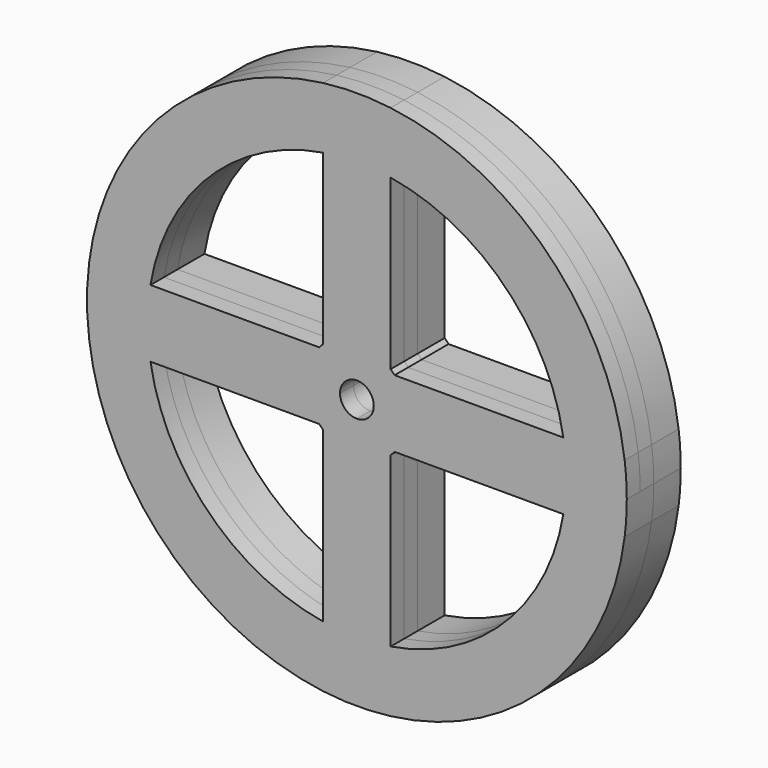
from build123d import *

# Parameters (mm, degrees)
F1_DEPTH = 2.5
F2_DEPTH = 5


# Not quite as in the source:
# - a feature names something its author has since deleted; it is built from what else it names


with BuildPart() as f1:
    # F0 (on Front) → F1 (new body, symmetric)
    with BuildSketch(Plane.XZ):
        with BuildLine():
            ThreePointArc((39.686269666, -5), (39.9214903695, -2.5049165017), (40, 0))
            ThreePointArc((40, 0), (39.9214903695, 2.5049165017), (39.686269666, 5))
            ThreePointArc((39.686269666, 5), (28.2842712475, 28.2842712475), (5, 39.686269666))
            ThreePointArc((5, 39.686269666), (0, 40), (-5, 39.686269666))
            ThreePointArc((-5, 39.686269666), (-28.2842712475, 28.2842712475), (-39.686269666, 5))
            ThreePointArc((-39.686269666, 5), (-40, 0), (-39.686269666, -5))
            ThreePointArc((-39.686269666, -5), (-28.2842712475, -28.2842712475), (-5, -39.686269666))
            ThreePointArc((-5, -39.686269666), (0, -40), (5, -39.686269666))
            ThreePointArc((5, -39.686269666), (28.2842712475, -28.2842712475), (39.686269666, -5))
        make_face()
        with BuildLine():
            ThreePointArc((30.5941170816, 5), (30.8983626551, 2.5082235219), (31, 0))
            ThreePointArc((31, 0), (30.8983626551, -2.5082235219), (30.5941170816, -5))
            ThreePointArc((30.5941170816, -5), (21.9203102168, -21.9203102168), (5, -30.5941170816))
            ThreePointArc((5, -30.5941170816), (2.5082235219, -30.8983626551), (0, -31))
            ThreePointArc((0, -31), (-2.5082235219, -30.8983626551), (-5, -30.5941170816))
            ThreePointArc((-5, -30.5941170816), (-21.9203102168, -21.9203102168), (-30.5941170816, -5))
            ThreePointArc((-30.5941170816, -5), (-30.8983626551, -2.5082235219), (-31, 0))
            ThreePointArc((-31, 0), (-30.8983626551, 2.5082235219), (-30.5941170816, 5))
            ThreePointArc((-30.5941170816, 5), (-21.9203102168, 21.9203102168), (-5, 30.5941170816))
            ThreePointArc((-5, 30.5941170816), (-2.5082235219, 30.8983626551), (0, 31))
            ThreePointArc((0, 31), (2.5082235219, 30.8983626551), (5, 30.5941170816))
            ThreePointArc((5, 30.5941170816), (21.9203102168, 21.9203102168), (30.5941170816, 5))
        make_face(mode=Mode.SUBTRACT)
        with BuildLine():
            Line((7.5, 0), (31, 0))
            ThreePointArc((31, 0), (30.8983626551, 2.5082235219), (30.5941170816, 5))
            Line((30.5941170816, 5), (5.5901699437, 5))
            ThreePointArc((5.5901699437, 5), (7.0062926922, 2.6761656733), (7.5, 0))
        make_face()
        with BuildLine():
            ThreePointArc((30.5941170816, -5), (30.8983626551, -2.5082235219), (31, 0))
            Line((31, 0), (7.5, 0))
            ThreePointArc((7.5, 0), (7.0062926922, -2.6761656733), (5.5901699437, -5))
            Line((5.5901699437, -5), (30.5941170816, -5))
        make_face()
        with BuildLine():
            Line((2.5, 0), (7.5, 0))
            ThreePointArc((7.5, 0), (7.0062926922, 2.6761656733), (5.5901699437, 5))
            ThreePointArc((5.5901699437, 5), (5.3033008589, 5.3033008589), (5, 5.5901699437))
            ThreePointArc((5, 5.5901699437), (2.6761656733, 7.0062926922), (0, 7.5))
            Line((0, 7.5), (0, 2.5))
            ThreePointArc((0, 2.5), (1.767766953, 1.767766953), (2.5, 0))
        make_face()
        with BuildLine():
            ThreePointArc((5.5901699437, -5), (7.0062926922, -2.6761656733), (7.5, 0))
            Line((7.5, 0), (2.5, 0))
            ThreePointArc((2.5, 0), (1.767766953, -1.767766953), (0, -2.5))
            Line((0, -2.5), (0, -7.5))
            ThreePointArc((0, -7.5), (2.6761656733, -7.0062926922), (5, -5.5901699437))
            ThreePointArc((5, -5.5901699437), (5.3033008589, -5.3033008589), (5.5901699437, -5))
        make_face()
        with BuildLine():
            Line((5, 5.5901699437), (5, 30.5941170816))
            ThreePointArc((5, 30.5941170816), (2.5082235219, 30.8983626551), (0, 31))
            Line((0, 31), (0, 7.5))
            ThreePointArc((0, 7.5), (2.6761656733, 7.0062926922), (5, 5.5901699437))
        make_face()
        with BuildLine():
            ThreePointArc((0, -31), (2.5082235219, -30.8983626551), (5, -30.5941170816))
            Line((5, -30.5941170816), (5, -5.5901699437))
            ThreePointArc((5, -5.5901699437), (2.6761656733, -7.0062926922), (0, -7.5))
            Line((0, -7.5), (0, -31))
        make_face()
        with BuildLine():
            Line((0, 7.5), (0, 31))
            ThreePointArc((0, 31), (-2.5082235219, 30.8983626551), (-5, 30.5941170816))
            Line((-5, 30.5941170816), (-5, 5.5901699437))
            ThreePointArc((-5, 5.5901699437), (-2.6761656733, 7.0062926922), (0, 7.5))
        make_face()
        with BuildLine():
            ThreePointArc((-5, -30.5941170816), (-2.5082235219, -30.8983626551), (0, -31))
            Line((0, -31), (0, -7.5))
            ThreePointArc((0, -7.5), (-2.6761656733, -7.0062926922), (-5, -5.5901699437))
            Line((-5, -5.5901699437), (-5, -30.5941170816))
        make_face()
        with BuildLine():
            ThreePointArc((-2.5, 0), (-1.767766953, 1.767766953), (0, 2.5))
            Line((0, 2.5), (0, 7.5))
            ThreePointArc((0, 7.5), (-2.6761656733, 7.0062926922), (-5, 5.5901699437))
            ThreePointArc((-5, 5.5901699437), (-5.3033008589, 5.3033008589), (-5.5901699437, 5))
            ThreePointArc((-5.5901699437, 5), (-7.0062926922, 2.6761656733), (-7.5, 0))
            Line((-7.5, 0), (-2.5, 0))
        make_face()
        with BuildLine():
            Line((0, -7.5), (0, -2.5))
            ThreePointArc((0, -2.5), (-1.767766953, -1.767766953), (-2.5, 0))
            Line((-2.5, 0), (-7.5, 0))
            ThreePointArc((-7.5, 0), (-7.0062926922, -2.6761656733), (-5.5901699437, -5))
            ThreePointArc((-5.5901699437, -5), (-5.3033008589, -5.3033008589), (-5, -5.5901699437))
            ThreePointArc((-5, -5.5901699437), (-2.6761656733, -7.0062926922), (0, -7.5))
        make_face()
        with BuildLine():
            Line((-5.5901699437, 5), (-30.5941170816, 5))
            ThreePointArc((-30.5941170816, 5), (-30.8983626551, 2.5082235219), (-31, 0))
            Line((-31, 0), (-7.5, 0))
            ThreePointArc((-7.5, 0), (-7.0062926922, 2.6761656733), (-5.5901699437, 5))
        make_face()
        with BuildLine():
            ThreePointArc((-31, 0), (-30.8983626551, -2.5082235219), (-30.5941170816, -5))
            Line((-30.5941170816, -5), (-5.5901699437, -5))
            ThreePointArc((-5.5901699437, -5), (-7.0062926922, -2.6761656733), (-7.5, 0))
            Line((-7.5, 0), (-31, 0))
        make_face()
    extrude(amount=F1_DEPTH, both=True)

    # F2 (add): a face of the model
    f2_faces = [f1.faces().sort_by_distance(p)[0] for p in [
        (-38.5637724499, 2.5, 4.8585786438),
    ]]
    extrude(f2_faces, amount=F2_DEPTH)


solid = f1.part
